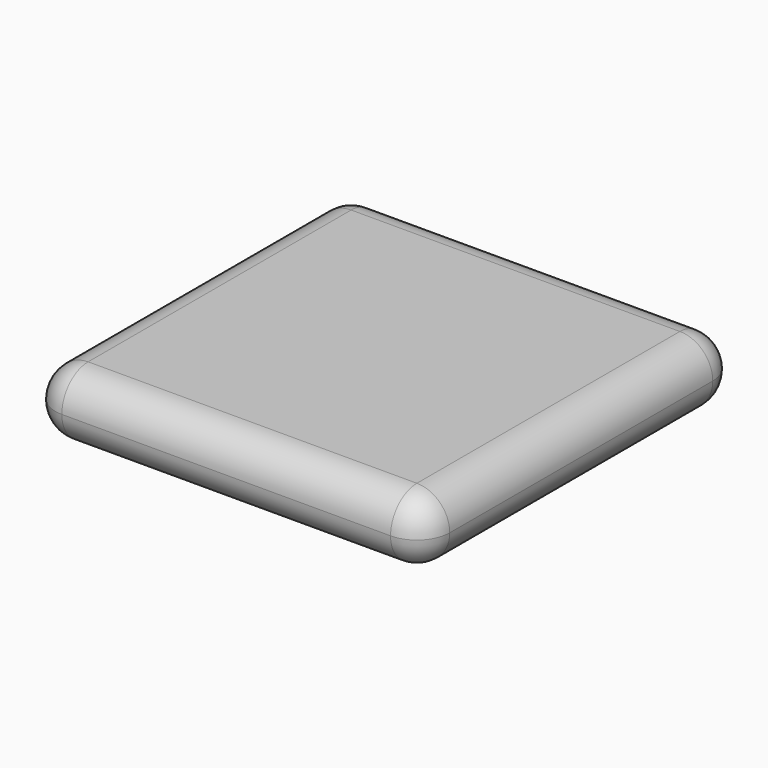
from build123d import *

# Parameters (mm, degrees)
F0_W     = 60
F0_H     = 60
F1_DEPTH = 10
F2_R     = 4.99999


# Not quite as in the source:
# - a fillet or chamfer is up to 0.001 mm smaller than in the source, because OpenCascade refuses the exact size


with BuildPart() as f1:
    # F0 (on Top) → F1 (new body)
    with BuildSketch(Plane.XY):
        with Locations((1.3857496455, 11.266246149)):
            Rectangle(F0_W, F0_H)
    extrude(amount=F1_DEPTH)

    # F2 (radius 5 in the source; OpenCascade refuses exactly that, so slightly less here)
    f2_edges = [f1.edges().sort_by_distance(p)[0] for p in [
        (-28.61425, 41.266246, 5),
        (-28.61425, -18.733754, 5),
        (-28.61425, 11.266246, 0),
        (-28.61425, 11.266246, 10),
        (31.38575, 41.266246, 5),
        (1.38575, 41.266246, 0),
        (1.38575, 41.266246, 10),
        (31.38575, -18.733754, 5),
        (1.38575, -18.733754, 0),
        (1.38575, -18.733754, 10),
        (31.38575, 11.266246, 0),
        (31.38575, 11.266246, 10),
    ]]
    fillet(f2_edges, radius=F2_R)


solid = f1.part
